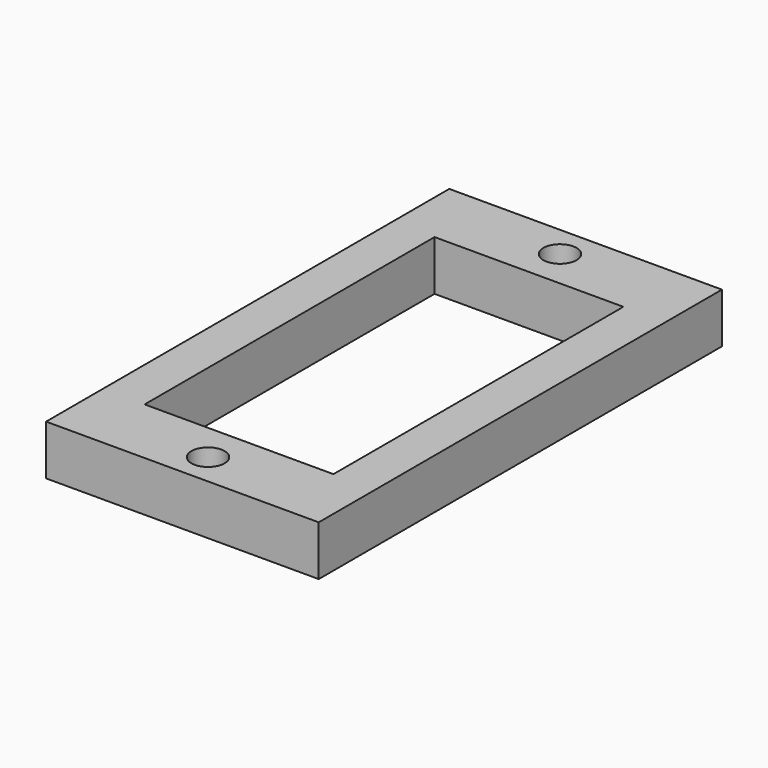
from build123d import *

# Parameters (mm, degrees)
F0_W     = 17.3136392439
F0_H     = 32.004
F0_R     = 1.0541
F0_W_2   = 11.9888
F0_H_2   = 23.0124
F1_DEPTH = 3.175


# Not quite as in the source:
# - a length typed as a fraction of an inch, garbled in the dataset ("3 / 203.2 mm" for 3/8 in), is restored


with BuildPart() as f1:
    # F0 (on Top) → F1 (new body)
    with BuildSketch(Plane.XY):
        Rectangle(F0_W, F0_H)
        with Locations((0, -13.97)):
            Circle(F0_R, mode=Mode.SUBTRACT)
        Rectangle(F0_W_2, F0_H_2, mode=Mode.SUBTRACT)
        with Locations((0, 13.97)):
            Circle(F0_R, mode=Mode.SUBTRACT)
    extrude(amount=F1_DEPTH)


solid = f1.part
